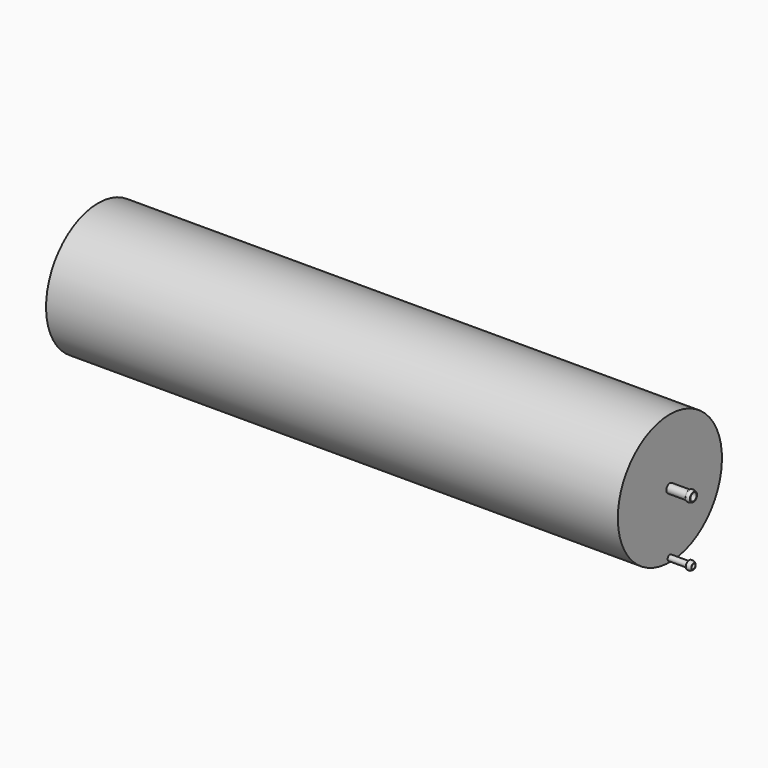
from build123d import *

# Parameters (mm, degrees)
F0_W     = 6
F0_H     = 190.6
F2_R     = 14.4
F3_DEPTH = 25.4
F4_R     = 9
F4_R_2   = 7.5
F5_DEPTH = 76.2


with BuildPart() as f1:
    # F0 (on Front) → F1 (revolve)
    with BuildSketch(Plane.XZ):
        Polygon((0, 210), (-1844.802, 210), (-1844.802, 205), (-6, 205), (0, 205), align=None)
        with Locations((-3, 109.7)):
            Rectangle(F0_W, F0_H)
        Polygon((63.5, 14.4), (0, 14.4), (-6, 14.4), (-6, 12.5), (76.2, 12.5), (76.2, 14.4), align=None)
        with BuildLine():
            Line((63.5, 17.2816771819), (63.5, 14.4))
            Line((63.5, 14.4), (76.2, 14.4))
            ThreePointArc((76.2, 14.4), (70.1280356313, 17.0661849066), (63.5, 17.2816771819))
        make_face()
    revolve(axis=Axis((-922.401, 0, 0), (1, 0, 0)))

    # F2 (on face) → F3 (cut)
    with BuildSketch(Plane.YZ):
        with BuildLine():
            ThreePointArc((-6.16e-08, -205), (5.3033008371, -202.8033008807), (7.5, -197.5))
            ThreePointArc((7.5, -197.5), (-5.3033008371, -192.1966991193), (-6.16e-08, -205))
        make_face()
        Circle(F2_R)
    extrude(amount=-F3_DEPTH, mode=Mode.SUBTRACT)

    # F4 (on face) → F5 (join)
    with BuildSketch(Plane.YZ):
        with Locations((0, -197.5)):
            Circle(F4_R)
        with Locations((0, -197.5)):
            Circle(F4_R_2, mode=Mode.SUBTRACT)
    extrude(amount=F5_DEPTH)

    # F6 (on Front) → F7 (revolve)
    with BuildSketch(Plane.XZ):
        with BuildLine():
            Line((62.23, -183.8815485485), (62.23, -188.5))
            Line((62.23, -188.5), (76.2, -188.5))
            ThreePointArc((76.2, -188.5), (69.8706444415, -184.2075656287), (62.23, -183.8815485485))
        make_face()
    revolve(axis=Axis((38.1, 0, -197.5), (-1, 0, 0)))


solid = f1.part
